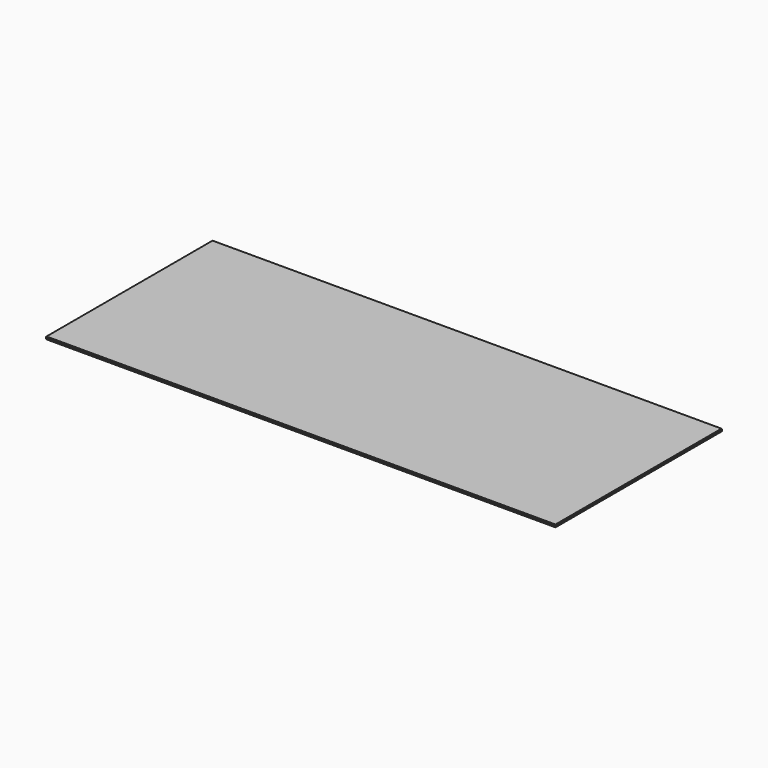
from build123d import *

# Parameters (mm, degrees)
F0_W     = 1184
F0_H     = 484
F1_DEPTH = 3
F2_SIZE  = 1
F3_SIZE  = 1
F4_SIZE  = 1
F5_SIZE  = 1
F6_SIZE  = 1
F7_SIZE  = 1


with BuildPart() as f1:
    # F0 (on Top) → F1 (new body, symmetric)
    with BuildSketch(Plane.XY):
        Rectangle(F0_W, F0_H)
    extrude(amount=F1_DEPTH, both=True)

    # F2
    f2_edges = [f1.edges().sort_by_distance(p)[0] for p in [
        (592, 0, -3),
        (0, -242, -3),
        (-592, 0, -3),
        (0, 242, -3),
    ]]
    chamfer(f2_edges, length=F2_SIZE)

    # F3
    f3_edges = [f1.edges().sort_by_distance(p)[0] for p in [
        (592, -242, 0.5),
    ]]
    chamfer(f3_edges, length=F3_SIZE)

    # F4
    f4_edges = [f1.edges().sort_by_distance(p)[0] for p in [
        (-592, 242, 0.5),
    ]]
    chamfer(f4_edges, length=F4_SIZE)

    # F5
    f5_edges = [f1.edges().sort_by_distance(p)[0] for p in [
        (-592, -242, 0.5),
    ]]
    chamfer(f5_edges, length=F5_SIZE)

    # F6
    f6_edges = [f1.edges().sort_by_distance(p)[0] for p in [
        (592, 242, 0.5),
    ]]
    chamfer(f6_edges, length=F6_SIZE)

    # F7 (call 1 of 4: OpenCascade refuses the feature's edges together)
    f7_edges = [f1.edges().sort_by_distance(p)[0] for p in [
        (0, -242, 3),
    ]]
    chamfer(f7_edges, length=F7_SIZE)

    # F7#2 (call 2 of 4)
    f7_2_edges = [f1.edges().sort_by_distance(p)[0] for p in [
        (592, 0, 3),
    ]]
    chamfer(f7_2_edges, length=F7_SIZE)

    # F7#3 (call 3 of 4)
    f7_3_edges = [f1.edges().sort_by_distance(p)[0] for p in [
        (0, 242, 3),
    ]]
    chamfer(f7_3_edges, length=F7_SIZE)

    # F7#4 (call 4 of 4)
    f7_4_edges = [f1.edges().sort_by_distance(p)[0] for p in [
        (-592, 0, 3),
    ]]
    chamfer(f7_4_edges, length=F7_SIZE)


solid = f1.part
